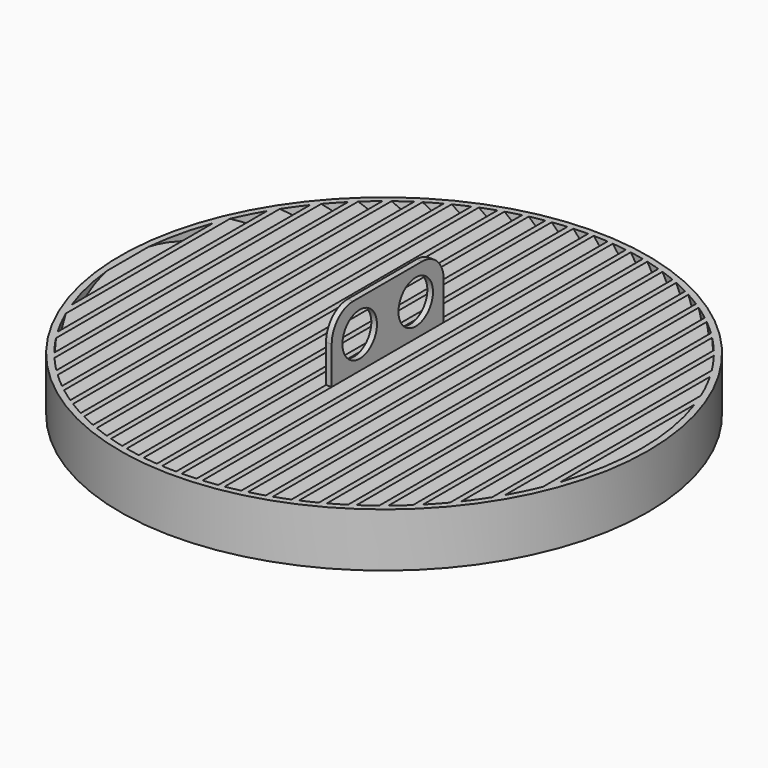
from build123d import *

# Parameters (mm, degrees)
F0_R     = 49
F0_R_2   = 47.8
F1_DEPTH = 10
F5_W     = 1.0443258315
F5_H     = 26
F6_DEPTH = 12
F8_DEPTH = 1.0443258315
F9_R     = 5


with BuildPart() as f1:
    # F0 (on Top) → F1 (new body)
    with BuildSketch(Plane.XY):
        Circle(F0_R)
        Circle(F0_R_2, mode=Mode.SUBTRACT)
    extrude(amount=F1_DEPTH)

    # F2 (on Front) → F3 (join, up to the next surface of F1)
    with BuildSketch(Plane.XZ):
        Polygon((-48.6, 3.6981042383), (-45.4969220976, 0), (-44.4525962661, 0), (-47.4729343578, 3.5994987715), (-44.3698564554, 6.203290295), (-47.5556741685, 10), (-48.6, 10), (-45.4969220976, 6.3018957617), align=None)
        Polygon((-41.7869220976, 0), (-40.7425962661, 0), (-43.7629343578, 3.5994987715), (-40.6598564554, 6.203290295), (-43.8456741685, 10), (-44.89, 10), (-41.7869220976, 6.3018957617), (-44.89, 3.6981042383), align=None)
        Polygon((-38.0769220976, 0), (-37.0325962661, 0), (-40.0529343578, 3.5994987715), (-36.9498564554, 6.203290295), (-40.1356741685, 10), (-41.18, 10), (-38.0769220976, 6.3018957617), (-41.18, 3.6981042383), align=None)
        Polygon((-34.3669220976, 0), (-33.3225962661, 0), (-36.3429343578, 3.5994987715), (-33.2398564554, 6.203290295), (-36.4256741685, 10), (-37.47, 10), (-34.3669220976, 6.3018957617), (-37.47, 3.6981042383), align=None)
        Polygon((-30.6569220976, 0), (-29.6125962661, 0), (-32.6329343578, 3.5994987715), (-29.5298564554, 6.203290295), (-32.7156741685, 10), (-33.76, 10), (-30.6569220976, 6.3018957617), (-33.76, 3.6981042383), align=None)
        Polygon((-26.9469220976, 0), (-25.9025962661, 0), (-28.9229343578, 3.5994987715), (-25.8198564554, 6.203290295), (-29.0056741685, 10), (-30.05, 10), (-26.9469220976, 6.3018957617), (-30.05, 3.6981042383), align=None)
        Polygon((-23.2369220976, 0), (-22.1925962661, 0), (-25.2129343578, 3.5994987715), (-22.1098564554, 6.203290295), (-25.2956741685, 10), (-26.34, 10), (-23.2369220976, 6.3018957617), (-26.34, 3.6981042383), align=None)
        Polygon((-19.5269220976, 0), (-18.4825962661, 0), (-21.5029343578, 3.5994987715), (-18.3998564554, 6.203290295), (-21.5856741685, 10), (-22.63, 10), (-19.5269220976, 6.3018957617), (-22.63, 3.6981042383), align=None)
        Polygon((-15.8169220976, 0), (-14.7725962661, 0), (-17.7929343578, 3.5994987715), (-14.6898564554, 6.203290295), (-17.8756741685, 10), (-18.92, 10), (-15.8169220976, 6.3018957617), (-18.92, 3.6981042383), align=None)
        Polygon((-12.1069220976, 0), (-11.0625962661, 0), (-14.0829343578, 3.5994987715), (-10.9798564554, 6.203290295), (-14.1656741685, 10), (-15.21, 10), (-12.1069220976, 6.3018957617), (-15.21, 3.6981042383), align=None)
        Polygon((-8.3969220976, 0), (-7.3525962661, 0), (-10.3729343578, 3.5994987715), (-7.2698564554, 6.203290295), (-10.4556741685, 10), (-11.5, 10), (-8.3969220976, 6.3018957617), (-11.5, 3.6981042383), align=None)
        Polygon((-4.6869220976, 0), (-3.6425962661, 0), (-6.6629343578, 3.5994987715), (-3.5598564554, 6.203290295), (-6.7456741685, 10), (-7.79, 10), (-4.6869220976, 6.3018957617), (-7.79, 3.6981042383), align=None)
        Polygon((-0.9769220976, 0), (0.0674037339, 0), (-2.9529343578, 3.5994987715), (0.1501435446, 6.203290295), (-3.0356741685, 10), (-4.08, 10), (-0.9769220976, 6.3018957617), (-4.08, 3.6981042383), align=None)
        Polygon((2.7330779024, 0), (3.7774037339, 0), (0.7570656422, 3.5994987715), (3.8601435446, 6.203290295), (0.6743258315, 10), (-0.37, 10), (2.7330779024, 6.3018957617), (-0.37, 3.6981042383), align=None)
        Polygon((6.4430779024, 0), (7.4874037339, 0), (4.4670656422, 3.5994987715), (7.5701435446, 6.203290295), (4.3843258315, 10), (3.34, 10), (6.4430779024, 6.3018957617), (3.34, 3.6981042383), align=None)
        Polygon((10.1530779024, 0), (11.1974037339, 0), (8.1770656422, 3.5994987715), (11.2801435446, 6.203290295), (8.0943258315, 10), (7.05, 10), (10.1530779024, 6.3018957617), (7.05, 3.6981042383), align=None)
        Polygon((13.8630779024, 0), (14.9074037339, 0), (11.8870656422, 3.5994987715), (14.9901435446, 6.203290295), (11.8043258315, 10), (10.76, 10), (13.8630779024, 6.3018957617), (10.76, 3.6981042383), align=None)
        Polygon((17.5730779024, 0), (18.6174037339, 0), (15.5970656422, 3.5994987715), (18.7001435446, 6.203290295), (15.5143258315, 10), (14.47, 10), (17.5730779024, 6.3018957617), (14.47, 3.6981042383), align=None)
        Polygon((21.2830779024, 0), (22.3274037339, 0), (19.3070656422, 3.5994987715), (22.4101435446, 6.203290295), (19.2243258315, 10), (18.18, 10), (21.2830779024, 6.3018957617), (18.18, 3.6981042383), align=None)
        Polygon((24.9930779024, 0), (26.0374037339, 0), (23.0170656422, 3.5994987715), (26.1201435446, 6.203290295), (22.9343258315, 10), (21.89, 10), (24.9930779024, 6.3018957617), (21.89, 3.6981042383), align=None)
        Polygon((28.7030779024, 0), (29.7474037339, 0), (26.7270656422, 3.5994987715), (29.8301435446, 6.203290295), (26.6443258315, 10), (25.6, 10), (28.7030779024, 6.3018957617), (25.6, 3.6981042383), align=None)
        Polygon((32.4130779024, 0), (33.4574037339, 0), (30.4370656422, 3.5994987715), (33.5401435446, 6.203290295), (30.3543258315, 10), (29.31, 10), (32.4130779024, 6.3018957617), (29.31, 3.6981042383), align=None)
        Polygon((36.1230779024, 0), (37.1674037339, 0), (34.1470656422, 3.5994987715), (37.2501435446, 6.203290295), (34.0643258315, 10), (33.02, 10), (36.1230779024, 6.3018957617), (33.02, 3.6981042383), align=None)
        Polygon((39.8330779024, 0), (40.8774037339, 0), (37.8570656422, 3.5994987715), (40.9601435446, 6.203290295), (37.7743258315, 10), (36.73, 10), (39.8330779024, 6.3018957617), (36.73, 3.6981042383), align=None)
        Polygon((43.5430779024, 0), (44.5874037339, 0), (41.5670656422, 3.5994987715), (44.6701435446, 6.203290295), (41.4843258315, 10), (40.44, 10), (43.5430779024, 6.3018957617), (40.44, 3.6981042383), align=None)
        Polygon((47.2530779024, 0), (48.2974037339, 0), (45.2770656422, 3.5994987715), (48.3801435446, 6.203290295), (45.1943258315, 10), (44.15, 10), (47.2530779024, 6.3018957617), (44.15, 3.6981042383), align=None)
    extrude(until=Until.NEXT, dir=(0, 1, 0))

    # F4: F1 across plane


with BuildPart() as f1_1:
    add(f1.part)
    add(f1.part.mirror(Plane.XZ))

    # F5 (on face) → F6 (join)
    with BuildSketch(Plane.XY.offset(10)):
        with Locations((0.1521629157, 0)):
            Rectangle(F5_W, F5_H)
    extrude(amount=F6_DEPTH)

    # F7 (on face) → F8 (cut, through all)
    with BuildSketch(Plane(origin=(-0.37, 0, 0), x_dir=(0, -1, 0), z_dir=(-1, 0, 0))):
        with BuildLine():
            add(Edge.make_bspline(
                [(-2.5, 16), (-2.5, 22.9282032303), (-8.5, 19.4641016151), (-14.5, 16), (-8.5, 12.5358983849), (-2.5, 9.0717967697), (-2.5, 16)],
                knots=[0, 0, 0, 2.0943951024, 2.0943951024, 4.1887902048, 4.1887902048, 6.2831853072, 6.2831853072, 6.2831853072], degree=2, weights=[1, 0.5, 1, 0.5, 1, 0.5, 1]))
        make_face()
        with BuildLine():
            add(Edge.make_bspline(
                [(10.5, 16), (10.5, 22.9282032303), (4.5, 19.4641016151), (-1.5, 16), (4.5, 12.5358983849), (10.5, 9.0717967697), (10.5, 16)],
                knots=[0, 0, 0, 2.0943951024, 2.0943951024, 4.1887902048, 4.1887902048, 6.2831853072, 6.2831853072, 6.2831853072], degree=2, weights=[1, 0.5, 1, 0.5, 1, 0.5, 1]))
        make_face()
    extrude(amount=-F8_DEPTH, mode=Mode.SUBTRACT)

    # F9
    f9_edges = [f1_1.edges().sort_by_distance(p)[0] for p in [
        (0.152163, 13, 22),
        (0.152163, -13, 22),
    ]]
    fillet(f9_edges, radius=F9_R)


solid = f1_1.part
